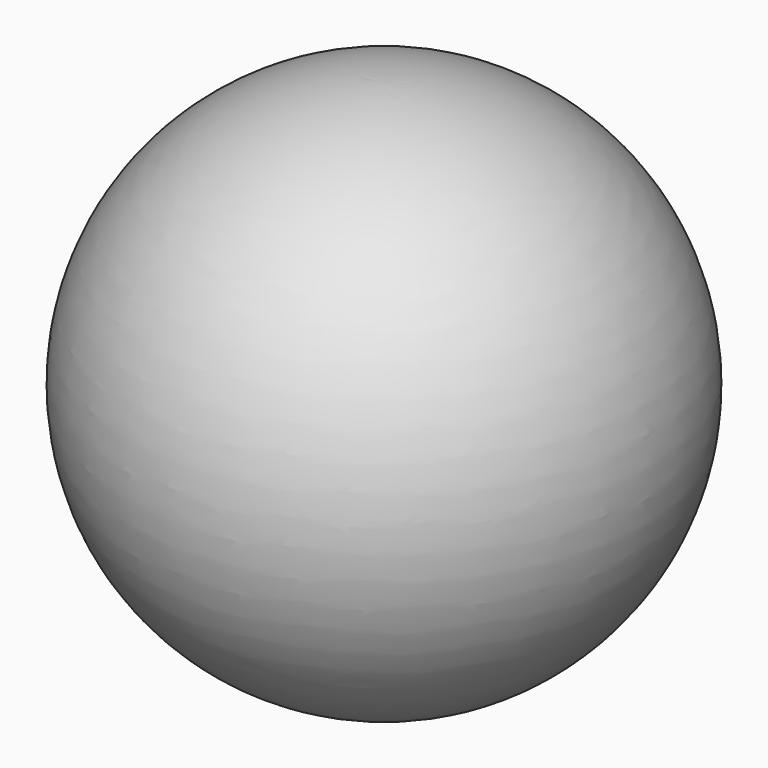
from build123d import *


with BuildPart() as f1:
    # F0 (on Front) → F1 (revolve)
    with BuildSketch(Plane.XZ):
        with BuildLine():
            Line((-0.3898801801, -50.7985038505), (0.0002633821, 50.7999999993))
            ThreePointArc((0.0002633821, 50.7999999993), (-50.7996254557, 0.1950732155), (-0.3898801801, -50.7985038505))
        make_face()
    revolve(axis=Axis((-0.194808399, 0, 0.0007480744), (-0.0038400239, 0, -0.9999926271)))


solid = f1.part
